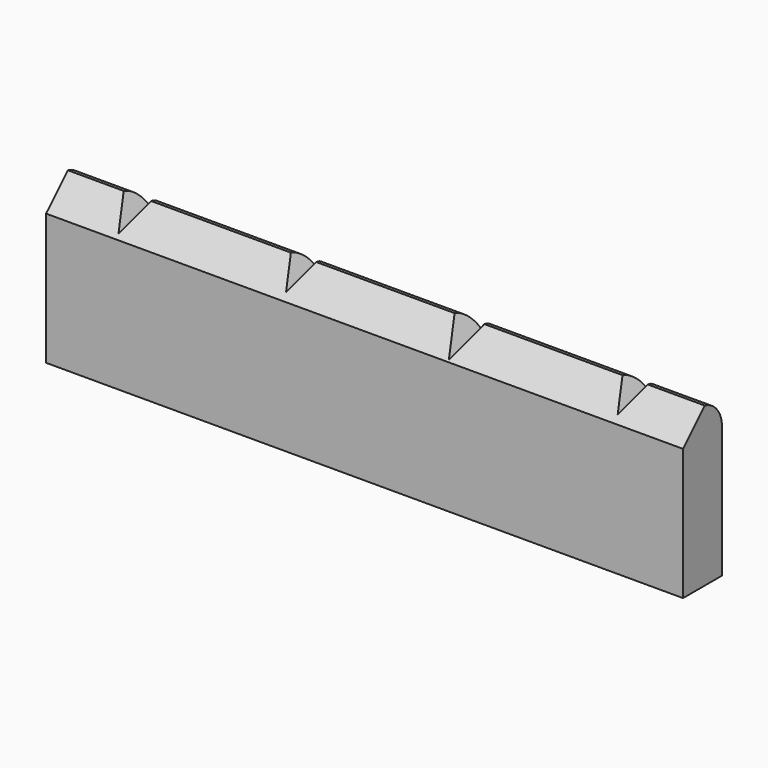
from build123d import *

# Parameters (mm, degrees)
F0_W        = 40.64
F0_H        = 3.0988
F1_DEPTH    = 10.16
F3_R        = 1.778
F4_T1_DEPTH = 49.7849047052
F5_DEPTH    = 25.4


# Not quite as in the source:
# - a fillet or chamfer that OpenCascade refuses, or shapes differently, is made with other operations: its cross-section is extruded or revolved along the edge and cut away or added


with BuildPart() as f1:
    # F0 (on Top) → F1 (new body)
    with BuildSketch(Plane.XY):
        with Locations((0, 1.5494)):
            Rectangle(F0_W, F0_H)
    extrude(amount=F1_DEPTH)

    # F3
    f3_edges = [f1.edges().sort_by_distance(p)[0] for p in [
        (0, 3.0988, 10.16),
    ]]
    fillet(f3_edges, radius=F3_R)

    # F4: chamfer of 1.778 on 1 edges, made by hand

    # F4_s2 → F4_t1 (cut)
    with BuildSketch(Plane.YZ.offset(-24.8924523526)):
        Polygon((1.778, 10.16), (0, 8.382), (0, 10.16), align=None)
    extrude(amount=F4_T1_DEPTH, mode=Mode.SUBTRACT)

    # F2 (on face) → F5 (cut)
    with BuildSketch(Plane.XZ):
        Polygon((-15.875, 8.5952954744), (-14.9716174209, 10.16), (-16.7783825791, 10.16), align=None)
        Polygon((-4.4531409051, 10.16), (-6.1132590949, 10.16), (-5.2832, 8.7222954744), align=None)
        Polygon((6.2853060633, 10.16), (4.3318939367, 10.16), (5.3086, 8.4682954744), align=None)
        Polygon((16.7050590949, 10.16), (15.0449409051, 10.16), (15.875, 8.7222954744), align=None)
    extrude(amount=-F5_DEPTH, mode=Mode.SUBTRACT)


solid = f1.part
